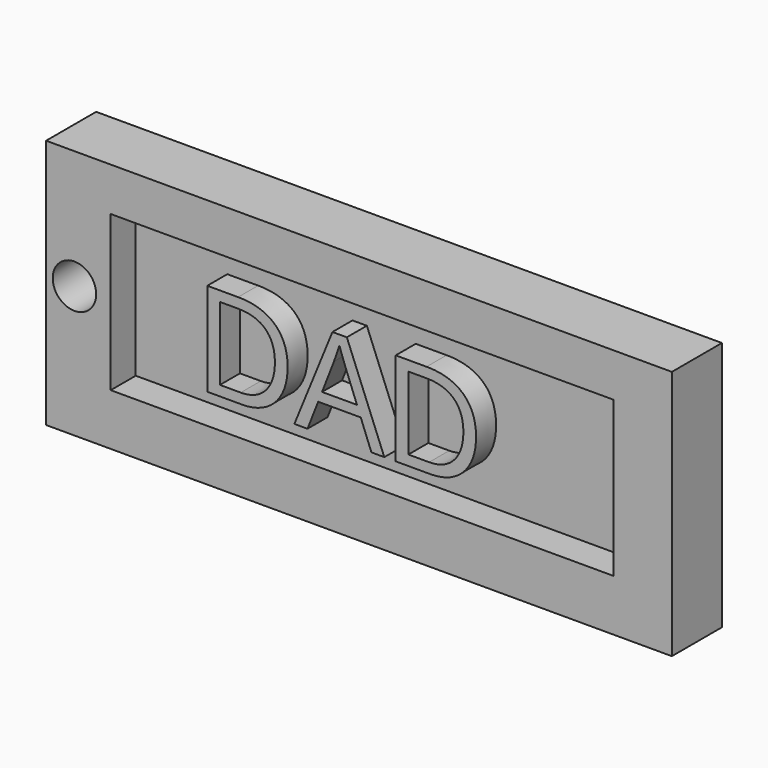
from build123d import *

# Parameters (mm, degrees)
F0_W         = 63.5
F0_H         = 25.4
F2_DEPTH     = 6.35
F3_W         = 51.0081909597
F3_H         = 15.739671886
F4_DEPTH     = 3.175
F5_R         = 2.2056472292
F6_DEPTH     = 12.7
F7_TEXT_SIZE = 13.7641172235
F8_DEPTH     = 2.54


# Not quite as in the source:
# - Text() gives the source's letters only with a copy of the font that has no kerning and outlines rounded to 1/6400 em; it was checked with that copy


with BuildPart() as f2:
    # F0 (on Front) → F2 (new body)
    with BuildSketch(Plane.XZ):
        with Locations((31.75, 12.7)):
            Rectangle(F0_W, F0_H)
    extrude(amount=F2_DEPTH)

    # F3 (on face) → F4 (cut)
    with BuildSketch(Plane.XZ.offset(6.35)):
        with Locations((32.0622939616, 13.1163932383)):
            Rectangle(F3_W, F3_H)
    extrude(amount=-F4_DEPTH, mode=Mode.SUBTRACT)

    # F5 (on Front) → F6 (cut, symmetric)
    with BuildSketch(Plane.XZ):
        with Locations((2.8792985249, 13.340132311)):
            Circle(F5_R)
    extrude(amount=F6_DEPTH, both=True, mode=Mode.SUBTRACT)

    # F7 (on face) → F8 (join)
    with BuildSketch(Plane.XZ.offset(3.175)):
        with Locations((14.7195095196, 7.869835943)):
            Text('DAD', F7_TEXT_SIZE, font='Arimo', text_align=(TextAlign.LEFT, TextAlign.BOTTOM))
    extrude(amount=F8_DEPTH)


solid = f2.part
